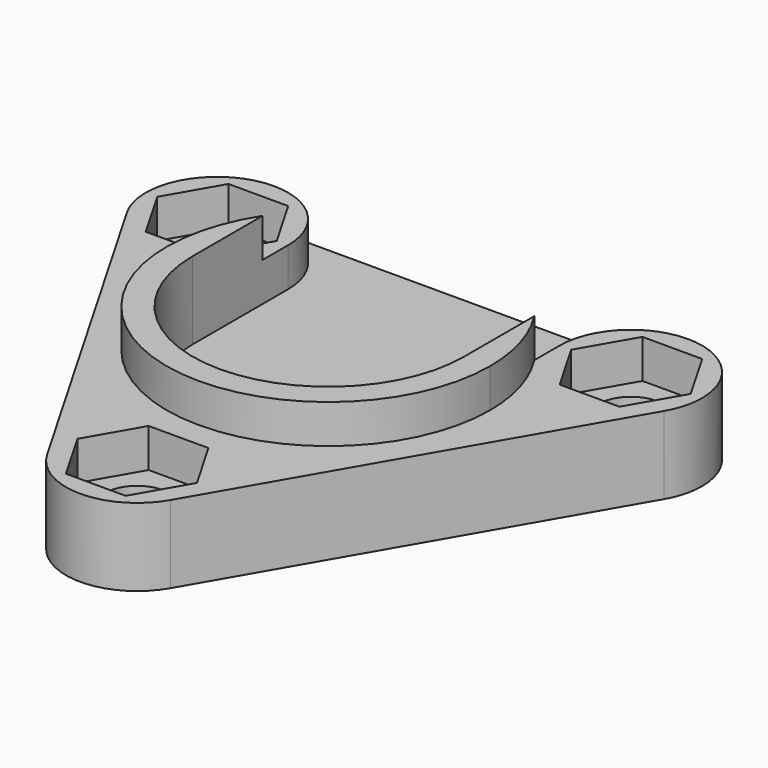
from build123d import *

# Parameters (mm, degrees)
F0_R     = 2.5
F1_DEPTH = 3
F2_START = 3
F2_DEPTH = 3
F3_START = 3
F3_DEPTH = 6


# Not quite as in the source:
# - a feature names something its author has since deleted; it is built from what else it names


with BuildPart() as f1:
    # F0 (on Top) → F1 (new body)
    with BuildSketch(Plane.XY):
        with BuildLine():
            ThreePointArc((-10.5, 0), (0, -10.5), (10.5, 0))
            ThreePointArc((10.5, 0), (0, 10.5), (-10.5, 0))
        make_face()
        with BuildLine():
            Line((10.5, 9.237604307), (10.5, 6.7823299831))
            ThreePointArc((10.5, 6.7823299831), (11.9895788083, 3.5355339059), (12.5, 0))
            ThreePointArc((12.5, 0), (-3.5355339059, -11.9895788083), (-10.5, 6.7823299831))
            Line((-10.5, 6.7823299831), (-10.5, 9.237604307))
            ThreePointArc((-10.5, 9.237604307), (-14.5764952519, 3.9250122624), (-20.7631397208, 6.487604307))
            Line((-20.7631397208, 6.487604307), (-4.7631397208, -21.2252086141))
            ThreePointArc((-4.7631397208, -21.2252086141), (-1.4235047481, -13.1626165695), (5.5, -18.4752086141))
            ThreePointArc((5.5, -18.4752086141), (5.3125920446, -19.8987133621), (4.7631397208, -21.2252086141))
            Line((4.7631397208, -21.2252086141), (20.7631397208, 6.487604307))
            ThreePointArc((20.7631397208, 6.487604307), (14.5764952519, 3.9250122624), (10.5, 9.237604307))
        make_face()
        with BuildLine():
            ThreePointArc((16, 14.737604307), (12.1109127035, 13.1266916036), (10.5, 9.237604307))
            ThreePointArc((10.5, 9.237604307), (14.5764952519, 3.9250122624), (20.7631397208, 6.487604307))
            ThreePointArc((20.7631397208, 6.487604307), (21.3125920446, 7.814099559), (21.5, 9.237604307))
            ThreePointArc((21.5, 9.237604307), (19.8890872965, 13.1266916036), (16, 14.737604307))
        make_face()
        Polygon((11.3811978465, 9.237604307), (13.6905989232, 13.237604307), (18.3094010768, 13.237604307), (20.6188021535, 9.237604307), (18.3094010768, 5.237604307), (13.6905989232, 5.237604307), align=None, mode=Mode.SUBTRACT)
        with BuildLine():
            ThreePointArc((-20.7631397208, 6.487604307), (-14.5764952519, 3.9250122624), (-10.5, 9.237604307))
            ThreePointArc((-10.5, 9.237604307), (-12.1109127035, 13.1266916036), (-16, 14.737604307))
            ThreePointArc((-16, 14.737604307), (-20.7631397208, 11.987604307), (-20.7631397208, 6.487604307))
        make_face()
        Polygon((-18.3094010768, 13.237604307), (-13.6905989232, 13.237604307), (-11.3811978465, 9.237604307), (-13.6905989232, 5.237604307), (-18.3094010768, 5.237604307), (-20.6188021535, 9.237604307), align=None, mode=Mode.SUBTRACT)
        with BuildLine():
            ThreePointArc((-4.7631397208, -21.2252086141), (0, -23.9752086141), (4.7631397208, -21.2252086141))
            ThreePointArc((4.7631397208, -21.2252086141), (5.3125920446, -19.8987133621), (5.5, -18.4752086141))
            ThreePointArc((5.5, -18.4752086141), (-1.4235047481, -13.1626165695), (-4.7631397208, -21.2252086141))
        make_face()
        Polygon((-2.3094010768, -22.4752086141), (-4.6188021535, -18.4752086141), (-2.3094010768, -14.4752086141), (2.3094010768, -14.4752086141), (4.6188021535, -18.4752086141), (2.3094010768, -22.4752086141), align=None, mode=Mode.SUBTRACT)
        with BuildLine():
            Line((10.5, 6.7823299831), (10.5, 0))
            ThreePointArc((10.5, 0), (0, -10.5), (-10.5, 0))
            Line((-10.5, 0), (-10.5, 6.7823299831))
            ThreePointArc((-10.5, 6.7823299831), (-3.5355339059, -11.9895788083), (12.5, 0))
            ThreePointArc((12.5, 0), (11.9895788083, 3.5355339059), (10.5, 6.7823299831))
        make_face()
        with BuildLine():
            ThreePointArc((-10.5, 6.7823299831), (0, 12.5), (10.5, 6.7823299831))
            Line((10.5, 6.7823299831), (10.5, 9.237604307))
            Line((10.5, 9.237604307), (10.5, 14.737604307))
            Line((10.5, 14.737604307), (-10.5, 14.737604307))
            Line((-10.5, 14.737604307), (-10.5, 9.237604307))
            Line((-10.5, 9.237604307), (-10.5, 6.7823299831))
        make_face()
        Polygon((18.3094010768, 13.237604307), (13.6905989232, 13.237604307), (11.3811978465, 9.237604307), (13.6905989232, 5.237604307), (18.3094010768, 5.237604307), (20.6188021535, 9.237604307), align=None)
        with Locations((16, 9.237604307)):
            Circle(F0_R, mode=Mode.SUBTRACT)
        Polygon((-2.3094010768, -14.4752086141), (-4.6188021535, -18.4752086141), (-2.3094010768, -22.4752086141), (2.3094010768, -22.4752086141), (4.6188021535, -18.4752086141), (2.3094010768, -14.4752086141), align=None)
        with Locations((0, -18.4752086141)):
            Circle(F0_R, mode=Mode.SUBTRACT)
        Polygon((-11.3811978465, 9.237604307), (-13.6905989232, 13.237604307), (-18.3094010768, 13.237604307), (-20.6188021535, 9.237604307), (-18.3094010768, 5.237604307), (-13.6905989232, 5.237604307), align=None)
        with Locations((-16, 9.237604307)):
            Circle(F0_R, mode=Mode.SUBTRACT)
        with BuildLine():
            ThreePointArc((-10.5, 0), (0, 10.5), (10.5, 0))
            Line((10.5, 0), (10.5, 6.7823299831))
            ThreePointArc((10.5, 6.7823299831), (0, 12.5), (-10.5, 6.7823299831))
            Line((-10.5, 6.7823299831), (-10.5, 0))
        make_face()
        with BuildLine():
            Line((10.5, 14.737604307), (10.5, 9.237604307))
            ThreePointArc((10.5, 9.237604307), (12.1109127035, 13.1266916036), (16, 14.737604307))
            Line((16, 14.737604307), (10.5, 14.737604307))
        make_face()
        with BuildLine():
            ThreePointArc((-16, 14.737604307), (-12.1109127035, 13.1266916036), (-10.5, 9.237604307))
            Line((-10.5, 9.237604307), (-10.5, 14.737604307))
            Line((-10.5, 14.737604307), (-16, 14.737604307))
        make_face()
    extrude(amount=F1_DEPTH)

    # F0 (on Top) → F2 (join)
    with BuildSketch(Plane.XY.offset(F2_START)):
        with BuildLine():
            ThreePointArc((-20.7631397208, 6.487604307), (-14.5764952519, 3.9250122624), (-10.5, 9.237604307))
            ThreePointArc((-10.5, 9.237604307), (-12.1109127035, 13.1266916036), (-16, 14.737604307))
            ThreePointArc((-16, 14.737604307), (-20.7631397208, 11.987604307), (-20.7631397208, 6.487604307))
        make_face()
        Polygon((-18.3094010768, 13.237604307), (-13.6905989232, 13.237604307), (-11.3811978465, 9.237604307), (-13.6905989232, 5.237604307), (-18.3094010768, 5.237604307), (-20.6188021535, 9.237604307), align=None, mode=Mode.SUBTRACT)
        with BuildLine():
            ThreePointArc((-4.7631397208, -21.2252086141), (0, -23.9752086141), (4.7631397208, -21.2252086141))
            ThreePointArc((4.7631397208, -21.2252086141), (5.3125920446, -19.8987133621), (5.5, -18.4752086141))
            ThreePointArc((5.5, -18.4752086141), (-1.4235047481, -13.1626165695), (-4.7631397208, -21.2252086141))
        make_face()
        Polygon((-2.3094010768, -22.4752086141), (-4.6188021535, -18.4752086141), (-2.3094010768, -14.4752086141), (2.3094010768, -14.4752086141), (4.6188021535, -18.4752086141), (2.3094010768, -22.4752086141), align=None, mode=Mode.SUBTRACT)
        with BuildLine():
            ThreePointArc((16, 14.737604307), (12.1109127035, 13.1266916036), (10.5, 9.237604307))
            ThreePointArc((10.5, 9.237604307), (14.5764952519, 3.9250122624), (20.7631397208, 6.487604307))
            ThreePointArc((20.7631397208, 6.487604307), (21.3125920446, 7.814099559), (21.5, 9.237604307))
            ThreePointArc((21.5, 9.237604307), (19.8890872965, 13.1266916036), (16, 14.737604307))
        make_face()
        Polygon((11.3811978465, 9.237604307), (13.6905989232, 13.237604307), (18.3094010768, 13.237604307), (20.6188021535, 9.237604307), (18.3094010768, 5.237604307), (13.6905989232, 5.237604307), align=None, mode=Mode.SUBTRACT)
        with BuildLine():
            Line((10.5, 9.237604307), (10.5, 6.7823299831))
            ThreePointArc((10.5, 6.7823299831), (11.9895788083, 3.5355339059), (12.5, 0))
            ThreePointArc((12.5, 0), (-3.5355339059, -11.9895788083), (-10.5, 6.7823299831))
            Line((-10.5, 6.7823299831), (-10.5, 9.237604307))
            ThreePointArc((-10.5, 9.237604307), (-14.5764952519, 3.9250122624), (-20.7631397208, 6.487604307))
            Line((-20.7631397208, 6.487604307), (-4.7631397208, -21.2252086141))
            ThreePointArc((-4.7631397208, -21.2252086141), (-1.4235047481, -13.1626165695), (5.5, -18.4752086141))
            ThreePointArc((5.5, -18.4752086141), (5.3125920446, -19.8987133621), (4.7631397208, -21.2252086141))
            Line((4.7631397208, -21.2252086141), (20.7631397208, 6.487604307))
            ThreePointArc((20.7631397208, 6.487604307), (14.5764952519, 3.9250122624), (10.5, 9.237604307))
        make_face()
    extrude(amount=F2_DEPTH)

    # F0 (on Top) → F3 (join)
    with BuildSketch(Plane.XY.offset(F3_START)):
        with BuildLine():
            Line((10.5, 6.7823299831), (10.5, 0))
            ThreePointArc((10.5, 0), (0, -10.5), (-10.5, 0))
            Line((-10.5, 0), (-10.5, 6.7823299831))
            ThreePointArc((-10.5, 6.7823299831), (-3.5355339059, -11.9895788083), (12.5, 0))
            ThreePointArc((12.5, 0), (11.9895788083, 3.5355339059), (10.5, 6.7823299831))
        make_face()
    extrude(amount=F3_DEPTH)


solid = f1.part
